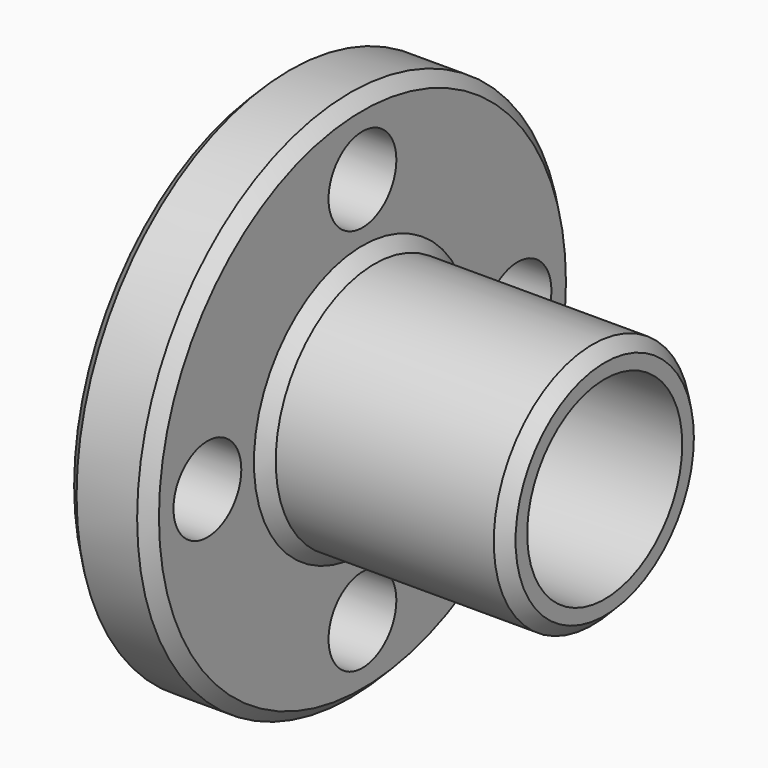
from build123d import *
from build123d import SkipClean  # not in build123d's __all__

# Parameters (mm, degrees)
F0_R      = 11
F1_DEPTH  = 3.5
F2_R      = 5.1
F3_DEPTH  = 10
F4_R      = 4
F5_DEPTH  = 25
F6_R      = 5.1
F6_R_2    = 4
F7_DEPTH  = 1.5
F8_SIZE   = 0.5
F9_R      = 1.75
F10_DEPTH = 5.001


# Not quite as in the source:
# - after a boolean that leaves OpenCascade's solid faulty, fix() repairs it


with BuildPart() as f1:
    # F0 (on Right) → F1 (new body)
    with BuildSketch(Plane.YZ):
        Circle(F0_R)
    extrude(amount=F1_DEPTH)

    # F2 (on face) → F3 (join)
    with BuildSketch(Plane.YZ.offset(3.5)):
        Circle(F2_R)
    extrude(amount=F3_DEPTH)

    # F4 (on face) → F5 (cut)
    with BuildSketch(Plane.YZ.offset(13.5)):
        Circle(F4_R)
    extrude(amount=-F5_DEPTH, mode=Mode.SUBTRACT)

    # F6 (on face) → F7 (join)
    with BuildSketch(Plane(origin=(0, 0, 0), x_dir=(0, -1, 0), z_dir=(-1, 0, 0))):
        Circle(F6_R)
        Circle(F6_R_2, mode=Mode.SUBTRACT)
    with SkipClean():  # cleaning this boolean's faces spoils the solid; the shape is the same uncleaned
        extrude(amount=F7_DEPTH)

    # F8
    f8_edges = [f1.edges().sort_by_distance(p)[0] for p in [
        (13.5, -5.1, 0),
        (3.5, -11, 0),
        (0, -11, 0),
        (-1.5, 5.1, 0),
        (3.5, -5.1, 0),
    ]]
    chamfer(f8_edges, length=F8_SIZE)

    # F9 (on face) → F10 (cut, through all)
    with BuildSketch(Plane.YZ.offset(3.5)):
        with Locations((0, 8)):
            Circle(F9_R)
        with Locations((-8, 0)):
            Circle(F9_R)
        with Locations((0, -8)):
            Circle(F9_R)
        with Locations((8, 0)):
            Circle(F9_R)
    extrude(amount=-F10_DEPTH, mode=Mode.SUBTRACT)

    add(f1.part.fix(), mode=Mode.REPLACE)


solid = f1.part
